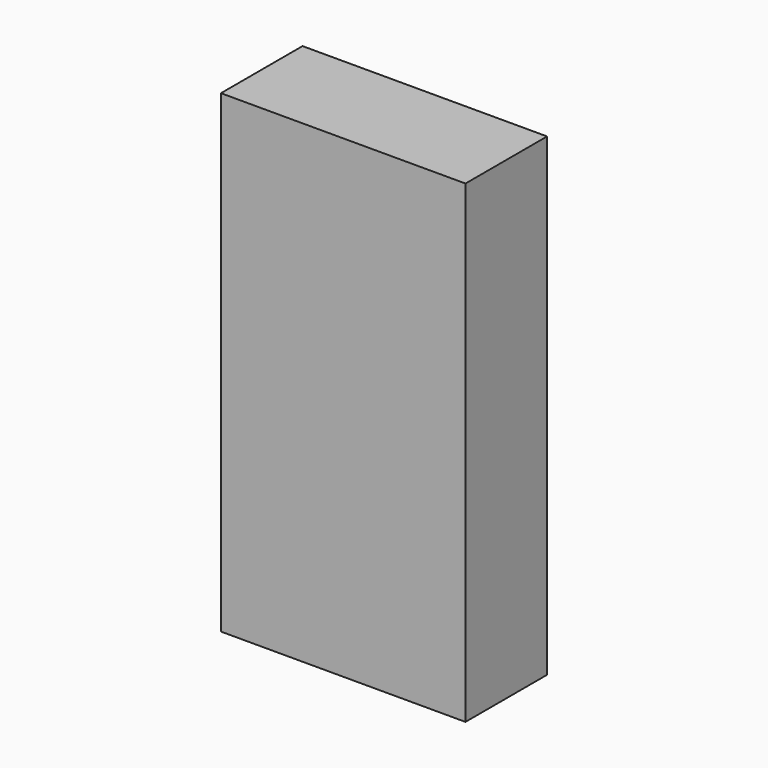
from build123d import *

# Parameters (mm, degrees)
F0_W     = 31.645745039
F0_H     = 13.1982266903
F1_DEPTH = 61.3355115056


# Not quite as in the source:
# - the program builds the solid bodies; features that only make, move or delete a surface that nothing else refers to are left out


with BuildPart() as f1:
    # F0 (on Top) → F1 (new body)
    with BuildSketch(Plane.XY):
        with Locations((-32.3206335306, 16.347810626)):
            Rectangle(F0_W, F0_H)
    extrude(amount=F1_DEPTH)


solid = f1.part
